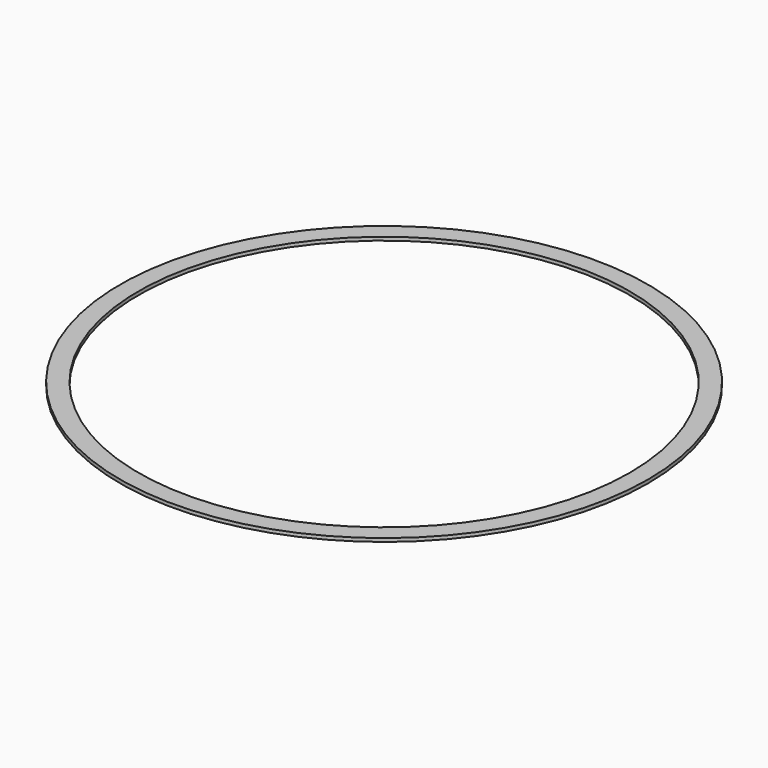
from build123d import *

# Parameters (mm, degrees)
F0_R     = 367.21161
F0_R_2   = 341.81161
F1_DEPTH = 4.7625


# Not quite as in the source:
# - a length typed as a fraction of an inch, garbled in the dataset ("3 / 203.2 mm" for 3/8 in), is restored


with BuildPart() as f1:
    # F0 (on Top) → F1 (new body)
    with BuildSketch(Plane.XY):
        Circle(F0_R)
        Circle(F0_R_2, mode=Mode.SUBTRACT)
    extrude(amount=F1_DEPTH)


solid = f1.part
